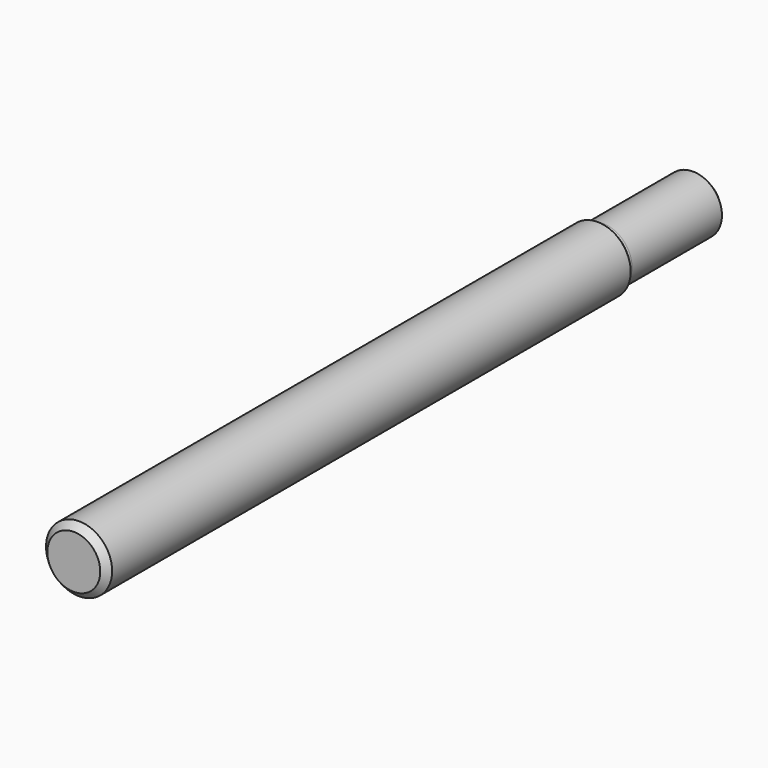
from build123d import *

# Parameters (mm, degrees)
F0_R        = 5
F1_DEPTH    = 100
F2_R        = 4.4
F3_DEPTH    = 18
F4_S5_R     = 4.4
F4_T6_DEPTH = 9
F5_SIZE     = 1


# Not quite as in the source:
# - a fillet or chamfer that OpenCascade refuses, or shapes differently, is made with other operations: its cross-section is extruded or revolved along the edge and cut away or added


with BuildPart() as f1:
    # F0 (on Front) → F1 (new body)
    with BuildSketch(Plane.XZ):
        Circle(F0_R)
    extrude(amount=F1_DEPTH)

    # F2 (on face) → F3 (join)
    with BuildSketch(Plane(origin=(0, 0, 0), x_dir=(-1, 0, 0), z_dir=(0, 1, 0))):
        Circle(F2_R)
    extrude(amount=F3_DEPTH)

    # F4: chamfer of 1 on 1 edges, made by hand


with BuildPart() as f4_tool2:
    # F4_s3 → F4_t4 (revolve)
    with BuildSketch(Plane.XY):
        Polygon((5, -1), (4, 0), (5, 0), align=None)
    revolve(axis=Axis((0, 0, 0), (0, -1, 0)))

    # F4_s5 → F4_t6 (cut, symmetric)
    with BuildSketch(Plane.XZ.offset(0.5)):
        Circle(F4_S5_R)
    extrude(amount=F4_T6_DEPTH, both=True, mode=Mode.SUBTRACT)


with BuildPart() as f1_1:
    add(f1.part)

    # F4_t1: cut F4_tool2
    add(f4_tool2.part, mode=Mode.SUBTRACT)

    # F5
    f5_edges = [f1_1.edges().sort_by_distance(p)[0] for p in [
        (-5, -100, 0),
        (4.4, 18, 0),
    ]]
    chamfer(f5_edges, length=F5_SIZE)


solid = f1_1.part
